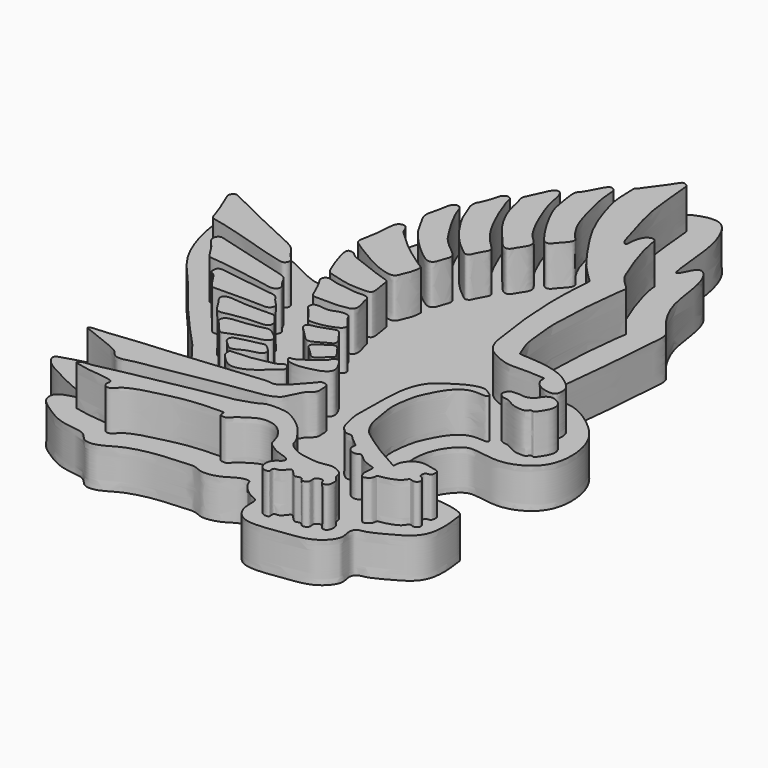
from build123d import *

# Parameters (mm, degrees)
F1_DEPTH     = 6.35
F3_DEPTH     = 6.35
F4_TEXT_SIZE = 5.2916666667
F5_DEPTH     = 3.175


# Not quite as in the source:
# - Text() gives the source's letters only with a copy of the font that has no kerning and outlines rounded to 1/6400 em; it was checked with that copy


with BuildPart() as f1:
    # F0 (on Top) → F1 (new body)
    with BuildSketch(Plane.XY):
        with BuildLine():
            add(Edge.make_bspline(
                [(-27.4553894997, -3.6191386171), (-26.8148858623, -4.1102651007), (-23.852993645, -3.5244667119), (-19.6757928123, -5.9814521208), (-16.3620676812, -9.2249197931), (-15.134802647, -13.3455814251), (-15.4166893319, -17.3130262849), (-17.4067311544, -20.0657025566), (-21.3949835552, -21.7431024541), (-25.6721295645, -20.6423826225), (-27.4943653261, -21.014570957), (-30.1702119684, -24.3150717379), (-30.2802703422, -29.5472485721), (-28.6378266919, -32.5947393842), (-24.4948659431, -36.2971740537), (-24.6097722846, -35.7640374591), (-22.7256148355, -34.3537072998), (-19.9838857156, -34.17260274), (-16.1665206622, -35.0662995786), (-16.01876004, -36.4181670777), (-15.67674916, -38.8146980995), (-15.8825278444, -43.0204957049), (-19.6794449856, -45.1478855127), (-22.3966423214, -46.5653511476), (-23.8193292554, -46.5918135896), (-24.3315319164, -47.8680905745), (-23.4823198149, -49.6082898374), (-25.9797320865, -52.64472308), (-30.6284736045, -52.9784109562), (-36.6825719823, -54.1169835226), (-38.7262257761, -50.7227346389), (-38.178485687, -48.1870624493), (-39.7768169823, -47.9738357147), (-42.0747997432, -45.9266069405), (-42.1528829746, -44.5168254865), (-44.2010819037, -44.9708731179), (-45.6685747061, -46.265967929), (-48.5542453701, -46.8428397062), (-49.8489739788, -45.940550258), (-51.6228374129, -46.0511790356), (-56.146626449, -46.3052263779), (-60.5609141609, -47.3991105071), (-62.9381972186, -49.2267616876), (-65.4295923454, -49.2927904494), (-66.3402420064, -47.2115411588), (-70.4619376248, -47.3761151768), (-73.6939821084, -45.2279395024), (-75.9213213355, -43.7444153615), (-76.1391517056, -41.6983734099), (-74.4737968942, -40.9017717278), (-72.7440822061, -40.6254899438), (-73.5010226256, -39.3395362954), (-76.0868419464, -38.415358059), (-78.7466419035, -37.0181314637), (-81.509071455, -35.6219927692), (-82.5651907032, -33.8226246448), (-80.9983905465, -33.3037701567), (-77.5024751636, -32.254660401), (-72.4511735406, -31.4168103779), (-67.3716768937, -30.6242442583), (-61.6508699498, -30.1812119822), (-61.7417475551, -29.6456508926), (-63.6792790879, -28.7025388346), (-66.8723911155, -26.0842687498), (-70.2278120042, -20.9467909755), (-73.9013952401, -17.3307431856), (-77.8419546016, -12.7167214029), (-81.8910703294, -7.3715338731), (-86.6721431792, -2.5965176686), (-88.9036740965, 4.918714181), (-88.8127902387, 8.3216580903), (-86.3142483502, 9.6224031711), (-82.2236034861, 8.0177620985), (-77.3124733662, 5.7624700254), (-72.4527478379, 3.3357110176), (-69.2384876898, 1.8166866233), (-67.2700148696, 2.21250367), (-68.0858159555, 5.2728469546), (-66.9871767241, 15.5792365266), (-62.6319303168, 26.3777930058), (-55.6842905211, 34.5100271747), (-49.290789682, 41.2499895243), (-44.4136194721, 45.7688665862), (-40.2069498195, 46.4674079992), (-38.2032900339, 44.1761388267), (-36.5613960949, 39.3943156931), (-36.303897104, 31.6116558315), (-35.3991681833, 32.1978806145), (-34.3181016042, 35.4947992226), (-31.4725448683, 32.2556409674), (-31.4109800539, 25.001298032), (-28.3660116525, 20.3349730668), (-26.8568790063, 18.7990546265), (-26.1921148547, 17.6879870326), (-26.6966478826, 14.2454097072), (-26.9886248875, 7.4933321266), (-27.9702700223, 0.0059592108), (-28.0853048722, -3.1361310215), (-27.4553894997, -3.6191386171)],
                knots=[0, 0, 0, 0, 0.0102621916, 0.0227218197, 0.0348262991, 0.0463747981, 0.057411536, 0.0674874786, 0.0790393719, 0.090657883, 0.0979966659, 0.1091456486, 0.121681532, 0.1330577825, 0.145274568, 0.1473172661, 0.1553303702, 0.165306988, 0.1759270057, 0.1817842271, 0.1905518788, 0.2017402263, 0.2132683224, 0.223194592, 0.2294367437, 0.2352939745, 0.242669919, 0.2528415109, 0.2653015886, 0.2788250284, 0.289029544, 0.2972399684, 0.3036406236, 0.3134592332, 0.3193121223, 0.3264488909, 0.3347261295, 0.344060323, 0.3508013577, 0.358032055, 0.3701207994, 0.3823246692, 0.3920357684, 0.4001190012, 0.407742519, 0.4186987314, 0.4299985352, 0.4390559444, 0.4461638099, 0.4536063147, 0.4602665683, 0.4656710985, 0.475032247, 0.485122963, 0.4951966568, 0.5021544279, 0.5082212727, 0.5190921769, 0.53186903, 0.5456635737, 0.5583206343, 0.5606866931, 0.5684030459, 0.5801350725, 0.5941202994, 0.6070219287, 0.620874169, 0.6354901951, 0.6503437704, 0.6660305311, 0.6758093578, 0.684132537, 0.695689388, 0.709120467, 0.7224849194, 0.7330496428, 0.7395731425, 0.7483200548, 0.766449771, 0.7860532177, 0.8045068132, 0.8218530155, 0.8363389009, 0.8470660296, 0.855966461, 0.8695152216, 0.8842974, 0.8878355848, 0.8969074862, 0.9060257583, 0.9216498602, 0.9348900886, 0.9428624087, 0.9487836087, 0.9588296365, 0.9738768003, 0.9899074542, 1, 1, 1, 1], degree=3))
        make_face()
    extrude(amount=-F1_DEPTH)

    # F2 (on Top) → F3 (join)
    with BuildSketch(Plane.XY):
        with BuildLine():
            add(Edge.make_bspline(
                [(-51.0431602597, -25.3127384931), (-51.2745821125, -25.3537660897), (-51.585693366, -25.239255998), (-51.5787417257, -25.7320025318), (-51.0000741928, -26.1592512167), (-50.2883419739, -26.4066127401), (-48.816850342, -26.3642354669), (-47.1832319042, -25.99359218), (-45.9112985427, -25.6087092918), (-45.0409266593, -24.8374675899), (-45.1042588573, -23.987436465), (-45.5408711668, -23.096610778), (-46.0647671328, -22.2476824891), (-46.4320555822, -21.9090460337), (-47.2162788837, -22.1575464864), (-47.2721777337, -22.7723006473), (-48.1069895995, -23.3821565507), (-49.2131278523, -24.2342290478), (-50.5653879125, -25.2280366774), (-51.0431602597, -25.3127384931)],
                knots=[0, 0, 0, 0, 0.0424248728, 0.0759988598, 0.1263997239, 0.1793440747, 0.252698589, 0.3328922948, 0.4037825364, 0.4660464316, 0.5191360524, 0.580846145, 0.6417531109, 0.6825286994, 0.7324827408, 0.7773888863, 0.8363898914, 0.9124134958, 1, 1, 1, 1], degree=3))
        make_face()
        with BuildLine():
            add(Edge.make_bspline(
                [(-50.4528097808, -22.5943885744), (-50.2009072172, -22.852652467), (-49.8842219204, -23.2714485333), (-49.3902502199, -23.4402195481), (-48.8550456144, -23.2750659834), (-48.2201713559, -22.5730329172), (-47.8716591404, -22.1185440384), (-47.41584488, -21.9220884176), (-47.1480308463, -21.436422456), (-47.8219759131, -20.5732866948), (-48.4205290406, -19.6615883887), (-48.9040339159, -19.2422247347), (-49.4735887631, -19.2412667677), (-51.0267468162, -20.4093166766), (-51.5230657887, -20.649471132), (-51.7808013374, -21.241737038), (-51.4194166847, -21.7362188103), (-50.757488413, -22.2820158521), (-50.4528097808, -22.5943885744)],
                knots=[0, 0, 0, 0, 0.0691757926, 0.118099141, 0.1706462329, 0.2412938083, 0.296871049, 0.3464913425, 0.3942791216, 0.468050598, 0.5464186234, 0.6011921627, 0.6531642032, 0.7537243571, 0.8100496669, 0.8621720635, 0.9163311974, 1, 1, 1, 1], degree=3))
        make_face()
        with BuildLine():
            add(Edge.make_bspline(
                [(-54.0498159826, -16.6909024119), (-54.4309451093, -16.7886579144), (-54.9236907464, -16.8100525559), (-55.4841457374, -17.150954382), (-55.5687185192, -17.7308079959), (-54.7835864349, -18.4822947196), (-53.6163201448, -19.6962753946), (-52.9839069298, -20.2793928352), (-52.3259906358, -20.3910920539), (-51.2503700733, -19.766276845), (-50.1447575111, -19.0834435117), (-49.5010374752, -18.9237958819), (-49.5203954014, -18.1112409278), (-50.1180495337, -17.3842322229), (-50.8593436979, -16.2880320165), (-51.2832647159, -15.8181698872), (-52.1847054864, -16.0003921099), (-53.4853314458, -16.5461182281), (-54.0498159826, -16.6909024119)],
                knots=[0, 0, 0, 0, 0.0623430111, 0.110971064, 0.1547311245, 0.2209242764, 0.306790441, 0.3657968767, 0.4145757926, 0.4865400119, 0.5618634321, 0.6100527431, 0.6615361337, 0.7258796456, 0.8007919939, 0.8486138498, 0.9076647171, 1, 1, 1, 1], degree=3))
        make_face()
        with BuildLine():
            add(Edge.make_bspline(
                [(-57.7154718339, -13.8489920646), (-57.4426548223, -14.1389097227), (-56.9641719318, -14.8565380209), (-56.286049579, -15.6886598531), (-55.9632417335, -16.0690516764), (-55.4678742171, -16.0825902786), (-53.8389666291, -16.0072877773), (-52.1807885496, -15.4218217794), (-51.3527076318, -14.9966475892), (-51.0961358405, -14.3577967622), (-51.5292296243, -13.8161515471), (-52.5457778427, -12.6549920363), (-52.7339673069, -11.9861971107), (-53.2393376369, -11.7540324128), (-54.2740386114, -11.6999497685), (-55.2828903014, -12.1988716378), (-56.294745799, -12.3544712206), (-57.359318583, -12.0967884211), (-58.1195223365, -12.2280027722), (-58.3442230508, -12.618076184), (-58.3730450927, -13.2826742755), (-57.9384009706, -13.6120893405), (-57.7154718339, -13.8489920646)],
                knots=[0, 0, 0, 0, 0.0607684619, 0.1166630656, 0.1521353154, 0.1872881217, 0.2557371584, 0.3285500365, 0.3791100111, 0.4186571539, 0.4619952422, 0.5291338699, 0.5726437839, 0.6097809741, 0.6635049593, 0.7205178734, 0.774489611, 0.8309049622, 0.8758032687, 0.9095722481, 0.950343783, 1, 1, 1, 1], degree=3))
        make_face()
        with BuildLine():
            add(Edge.make_bspline(
                [(-60.7358627021, -8.3436481655), (-60.5109025038, -8.8366568045), (-60.0222166665, -9.929884189), (-59.7570486348, -10.4844665724), (-58.9535402781, -10.6414034882), (-56.8626474343, -10.5041612494), (-55.6637065415, -10.6341358809), (-54.7588632897, -10.3865299306), (-53.9212650186, -10.3516184605), (-53.3479837532, -10.0031467426), (-53.3797547819, -8.7030940872), (-53.8434332345, -7.7117374992), (-53.8591402127, -6.9498398962), (-54.4305145001, -6.3020606164), (-56.0589847258, -6.5427869114), (-57.6440529799, -6.2479909036), (-59.3693243668, -6.0882031906), (-60.4773564804, -5.7059013677), (-61.1720251234, -5.4724937862), (-61.7435067891, -5.9118030363), (-61.8360537136, -6.5333694945), (-61.1522655527, -7.4480877708), (-60.9094500005, -7.9632251468), (-60.7358627021, -8.3436481655)],
                knots=[0, 0, 0, 0, 0.0624029211, 0.0974424366, 0.1372974836, 0.2058511483, 0.2583779573, 0.3030843904, 0.3456217278, 0.3807091631, 0.4320737739, 0.4821055108, 0.5218767272, 0.5611719847, 0.6194538937, 0.680689788, 0.7425669549, 0.793462225, 0.8318720338, 0.868564241, 0.9035233534, 0.9518476843, 1, 1, 1, 1], degree=3))
        make_face()
        with BuildLine():
            add(Edge.make_bspline(
                [(-63.1658956409, -1.7125232844), (-63.0045333751, -2.1921836237), (-62.4267597088, -3.619248892), (-62.0076478412, -4.3340511705), (-60.5316804198, -4.7342371742), (-58.3200695619, -5.3290594722), (-56.8862224099, -5.3724035497), (-55.1673104854, -5.443421827), (-54.3485208479, -5.1358791957), (-54.6817931828, -3.3548648601), (-54.864479756, -2.182940092), (-54.9692438631, -1.5676601204), (-56.3391111992, -1.2358353906), (-58.7053830333, -0.3204373165), (-60.8115823361, 0.4237868214), (-62.3934344299, 1.0489225409), (-62.8427436767, 1.7102418304), (-63.6170293643, 1.8040869196), (-63.9838731163, 1.6413681894), (-63.9428352401, 0.5020270597), (-63.3329459418, -1.0564756941), (-63.2621516745, -1.4263956598), (-63.1658956409, -1.7125232844)],
                knots=[0, 0, 0, 0, 0.0632553349, 0.1035080117, 0.1567836407, 0.2245909001, 0.2797039683, 0.3373897643, 0.3733866441, 0.4306452931, 0.480800148, 0.5119031271, 0.5615171308, 0.6339424884, 0.7023298543, 0.7588686609, 0.7974842832, 0.8347087637, 0.8591793167, 0.9047103225, 0.9622668433, 1, 1, 1, 1], degree=3))
        make_face()
        with BuildLine():
            add(Edge.make_bspline(
                [(-54.5166023076, 1.4176972909), (-54.6447443239, 1.0994388626), (-54.8698592937, 0.2716580084), (-55.5827005827, -0.2034733354), (-57.5127285564, 0.3038740625), (-59.4111238997, 1.1389104479), (-61.6868451024, 2.498020546), (-63.5273637309, 3.6024866333), (-64.2630764338, 4.1697785139), (-64.6025305916, 4.682970505), (-64.1201272309, 6.4661454363), (-63.8888361785, 8.6367543167), (-63.8404456098, 10.0627233024), (-63.6938059845, 10.9044395082), (-63.1964883809, 11.4137262798), (-62.4477548249, 11.4092981949), (-62.0200031326, 10.9287249345), (-61.788630202, 9.988860788), (-60.6421140061, 8.9994838577), (-58.2929077591, 6.7758939232), (-56.4615499088, 5.5470369783), (-54.2249516192, 3.943826605), (-53.8537274399, 3.860001145), (-54.1412079286, 2.0873732774), (-54.4060345119, 1.6923077104), (-54.5166023076, 1.4176972909)],
                knots=[0, 0, 0, 0, 0.0403213228, 0.0722907996, 0.123225953, 0.1786009007, 0.2402506999, 0.295383211, 0.3301347634, 0.3567284474, 0.406328799, 0.4634682132, 0.5080869031, 0.5417299103, 0.5717362827, 0.6021603181, 0.6307636117, 0.6660244815, 0.7118570167, 0.7785806429, 0.8384723649, 0.8982011422, 0.918092635, 0.9652086028, 1, 1, 1, 1], degree=3))
        make_face()
        with BuildLine():
            add(Edge.make_bspline(
                [(-53.1711541116, 7.1701635607), (-53.3105781169, 6.7492806406), (-53.4716730845, 5.9789526739), (-54.2863918399, 5.6005413816), (-55.4231005052, 6.2283311505), (-57.2882570655, 7.7624896831), (-59.5468859643, 10.0709520788), (-60.6654709352, 11.6820484836), (-61.7566180282, 13.7522765324), (-62.3966302917, 14.8764981582), (-62.3275485786, 15.977989267), (-61.9880298763, 16.9363475846), (-61.7731718938, 18.4349866598), (-61.569983331, 19.2516531435), (-61.0211940861, 19.7970319664), (-60.2066459209, 19.5275052108), (-59.9675942575, 18.7598000322), (-59.6092806702, 17.7060062264), (-58.3475878373, 15.2595831608), (-57.3093597118, 13.6623655769), (-56.1212070678, 11.63494563), (-54.39603909, 10.1563411757), (-53.0426019954, 9.1157164841), (-52.697914576, 8.3116263071), (-53.0320326557, 7.5901331671), (-53.1711541116, 7.1701635607)],
                knots=[0, 0, 0, 0, 0.039898997, 0.0702664358, 0.1092829888, 0.1666472165, 0.2319081805, 0.2837228223, 0.3386738763, 0.3797090762, 0.4160458165, 0.4532174902, 0.4977869395, 0.5312683359, 0.5606193333, 0.5910624073, 0.6219561444, 0.6605316435, 0.720323481, 0.7717601497, 0.8266202781, 0.882147647, 0.9288142546, 0.9601875836, 1, 1, 1, 1], degree=3))
        make_face()
        with BuildLine():
            add(Edge.make_bspline(
                [(-51.0917045176, 10.9392181039), (-50.9316985491, 11.3158911058), (-50.3528916686, 12.2805013852), (-50.1531429412, 12.6678430146), (-50.1812438653, 13.2395001883), (-50.7664969895, 13.7285995148), (-52.5108285766, 15.5683909941), (-54.0314576577, 17.9494110834), (-55.3060962907, 20.6428028672), (-56.4803985508, 23.6078114587), (-56.7334668006, 24.5797465807), (-56.7771196516, 25.1520674835), (-57.3520138011, 25.5892177215), (-58.216930852, 25.3002126115), (-58.3961059888, 24.1185147938), (-59.1377946686, 22.10096233), (-59.5553529504, 21.6305186663), (-59.5625931359, 20.534293305), (-59.0133823443, 19.5552161164), (-58.4417468898, 17.5616656282), (-56.8585294675, 15.0999632533), (-55.3395474196, 12.9655536672), (-53.569806434, 11.263160302), (-52.434838729, 10.4501372633), (-51.9004632146, 9.9596016167), (-51.2275285866, 10.4246897047), (-51.1889013683, 10.7104052049), (-51.0917045176, 10.9392181039)],
                knots=[0, 0, 0, 0, 0.0428191915, 0.0665158463, 0.0901826796, 0.1192645229, 0.1738998829, 0.2330867527, 0.2943581485, 0.3560382157, 0.3899960048, 0.4148468355, 0.4421371427, 0.4714925245, 0.5092073668, 0.5598807532, 0.5874582961, 0.6214236717, 0.6580905013, 0.7075789677, 0.7672274593, 0.8242719642, 0.8786200138, 0.9195011783, 0.9464068898, 0.9739891543, 1, 1, 1, 1], degree=3))
        make_face()
        with BuildLine():
            add(Edge.make_bspline(
                [(-47.9384362698, 15.4462410137), (-48.1485071319, 15.0888367792), (-48.439799129, 14.4005355663), (-49.5143881239, 14.4486574045), (-50.5872523186, 15.9064331362), (-52.7048998917, 18.1192732527), (-55.0535786663, 22.0368695313), (-55.5554723592, 25.3791421715), (-56.047950592, 26.3482300709), (-55.1830697963, 27.8480265522), (-54.4659959127, 29.8143455459), (-53.8584459064, 30.5158066731), (-53.1022762667, 30.581119463), (-52.5234780041, 29.3820377371), (-52.2673493499, 27.3033143389), (-51.3487014244, 24.7516881437), (-49.9692488311, 21.3690426082), (-48.4465691577, 18.9102443266), (-47.2231523777, 18.0050783015), (-47.0024361702, 17.2741434341), (-47.1933450462, 16.4949970442), (-47.708548397, 15.8373609357), (-47.9384362698, 15.4462410137)],
                knots=[0, 0, 0, 0, 0.039865054, 0.0738579514, 0.1231907968, 0.1907245817, 0.2736975541, 0.342631572, 0.3794403252, 0.4280645022, 0.4843416426, 0.5196037397, 0.5482098592, 0.589097779, 0.644576485, 0.7078489474, 0.7817048357, 0.8468647205, 0.8922445629, 0.9233351121, 0.9563742807, 1, 1, 1, 1], degree=3))
        make_face()
        with BuildLine():
            add(Edge.make_bspline(
                [(-44.8181889951, 19.6065697819), (-45.0892064683, 19.2871625125), (-45.3788242436, 18.7999570147), (-46.2986300849, 18.590227551), (-47.4578400977, 20.2381493905), (-48.8852804579, 22.3426059612), (-50.8161913432, 25.9981887098), (-51.1444078282, 27.884796994), (-51.8268805321, 31.5411972258), (-51.0618173958, 32.0335731457), (-50.0871851427, 33.9191341711), (-49.5800350058, 34.9476354883), (-49.0395552817, 35.5252647073), (-48.0908482922, 35.1087779939), (-48.1312390451, 33.8118591772), (-47.792653536, 31.1049486779), (-47.0194097064, 28.4879754833), (-46.0895843554, 24.6840873365), (-44.1677175413, 22.1645527023), (-43.6017539823, 21.6738521255), (-43.5545785906, 20.8678150492), (-44.4563897318, 20.0329678049), (-44.8181889951, 19.6065697819)],
                knots=[0, 0, 0, 0, 0.0378274782, 0.0691585245, 0.1195601458, 0.1829731268, 0.2583107602, 0.3149733325, 0.3842953787, 0.4185585686, 0.4729611357, 0.5149839133, 0.5455084659, 0.578607853, 0.6197428268, 0.6820513078, 0.7458440771, 0.8220643302, 0.8882718996, 0.9190368084, 0.9495015817, 1, 1, 1, 1], degree=3))
        make_face()
        with BuildLine():
            add(Edge.make_bspline(
                [(-52.1277524531, -27.7087949216), (-51.8088840319, -27.6149246016), (-51.286925511, -27.4192252053), (-50.9870676499, -27.0151117761), (-50.3096205755, -27.1869428315), (-49.8486741782, -28.1034559834), (-50.8239688554, -28.915458337), (-53.0422379923, -30.8232362152), (-54.5368178641, -31.505509584), (-56.3342580058, -31.7646219494), (-57.8074216971, -30.2967440914), (-58.5308978238, -29.5099387288), (-58.5333976199, -28.4641574981), (-58.0577588336, -28.5419980378), (-57.005444184, -28.4553344204), (-55.4182671766, -28.4078400516), (-53.4163705845, -28.0067200418), (-52.5125475895, -27.8220731274), (-52.1277524531, -27.7087949216)],
                knots=[0, 0, 0, 0, 0.0543149208, 0.0920882672, 0.1357996319, 0.1873570917, 0.2479667751, 0.3467624855, 0.4217089292, 0.4949345576, 0.5752045882, 0.6361262063, 0.6872002987, 0.7200634138, 0.7782354761, 0.8522042876, 0.9344553553, 1, 1, 1, 1], degree=3))
        make_face()
        with BuildLine():
            add(Edge.make_bspline(
                [(-59.1037757695, -27.8701167554), (-59.3867114578, -27.7586753043), (-59.9015092741, -27.1582175687), (-60.752400481, -26.5310875516), (-60.6486679325, -25.5186310355), (-59.7587590572, -25.3350527773), (-58.0999296109, -24.843394082), (-56.6078943641, -24.6179665266), (-56.0142146092, -24.335954542), (-54.8437192915, -25.3786490842), (-54.6154403266, -26.0301054732), (-55.0249652733, -26.7552581276), (-56.8976626709, -26.9520600961), (-58.2138886704, -27.8513727568), (-58.85678463, -27.9674005274), (-59.1037757695, -27.8701167554)],
                knots=[0, 0, 0, 0, 0.0764864722, 0.1521062383, 0.2170449898, 0.2828926781, 0.3829175026, 0.473739006, 0.5298584413, 0.6185554221, 0.6785568114, 0.7380386801, 0.8382194979, 0.9332304771, 1, 1, 1, 1], degree=3))
        make_face()
        with BuildLine():
            add(Edge.make_bspline(
                [(-64.1955733299, -23.5584191978), (-64.4168101868, -23.3225329439), (-64.8914748812, -22.8895621988), (-64.6162161632, -21.9752148969), (-63.5384869306, -21.639683951), (-62.0631338553, -21.6102629156), (-59.5317277557, -21.2198383227), (-58.2944643813, -20.805447507), (-57.5752089731, -21.2453764724), (-56.275804026, -22.2599392976), (-56.188069735, -23.0564824809), (-57.0851128872, -23.7105777497), (-58.2721813874, -23.7969972815), (-60.4757327663, -24.5644636684), (-61.9118511863, -25.1201866516), (-62.6279019718, -25.4661083664), (-63.5162139191, -24.3799194723), (-63.9494881965, -23.8207990792), (-64.1955733299, -23.5584191978)],
                knots=[0, 0, 0, 0, 0.0542836285, 0.1034632979, 0.1604990261, 0.2312516689, 0.323195176, 0.3857590257, 0.4364446556, 0.5086048249, 0.5544493793, 0.6095763308, 0.6724148373, 0.7599936256, 0.8313677159, 0.8764142381, 0.9396194912, 1, 1, 1, 1], degree=3))
        make_face()
        with BuildLine():
            add(Edge.make_bspline(
                [(-59.4865120947, -18.425444141), (-59.2638501523, -18.6830200711), (-58.8257997499, -19.0313878599), (-58.8116014315, -20.0025863892), (-59.3794496569, -20.4197684226), (-60.8016950369, -20.2884110893), (-64.4641465023, -20.7320199747), (-65.7044642864, -21.1557047885), (-66.7138447348, -21.0567343718), (-67.4807513994, -19.4746651997), (-68.309721875, -18.5362976168), (-68.4801477188, -17.8282118041), (-67.8498206622, -17.1734034611), (-65.9742048578, -17.5155911769), (-63.172923641, -17.6280361999), (-60.7868338767, -17.5369060919), (-60.143848462, -17.4995899714), (-59.7294264447, -18.1444401719), (-59.4865120947, -18.425444141)],
                knots=[0, 0, 0, 0, 0.0520802351, 0.1018697119, 0.1426877185, 0.2079163619, 0.31431348, 0.3777797851, 0.4273616376, 0.4986611868, 0.5612411578, 0.6041474294, 0.6496069169, 0.7228084543, 0.8188129076, 0.9024515806, 0.9431827625, 1, 1, 1, 1], degree=3))
        make_face()
        with BuildLine():
            add(Edge.make_bspline(
                [(-62.6528635621, -14.2897320911), (-62.3977079997, -14.6054204859), (-61.8006268013, -15.1674059642), (-61.497322134, -15.6402146615), (-61.8927338613, -16.5733610994), (-63.5119533205, -16.4274544566), (-67.6943494865, -16.4249644458), (-70.5294653786, -16.4981483154), (-70.9313768732, -16.4816516671), (-71.7635540579, -15.5852705442), (-72.849471562, -13.5195999757), (-73.7076458282, -13.524291081), (-73.6746109316, -12.3686058372), (-73.3505191838, -11.9918400504), (-72.0982646784, -12.0703922949), (-70.1896615181, -12.4356531572), (-67.546822934, -12.732640641), (-65.0660478183, -13.2275666342), (-63.838902823, -13.2188493763), (-63.1298621483, -13.555889556), (-62.8678978928, -14.0236832462), (-62.6528635621, -14.2897320911)],
                knots=[0, 0, 0, 0, 0.0509343677, 0.0839290619, 0.123384639, 0.1779115246, 0.2754749073, 0.3509697989, 0.3766312536, 0.4260584754, 0.4957413496, 0.5323748479, 0.5768002726, 0.6067240334, 0.6551090129, 0.7199823636, 0.7960430866, 0.8692766927, 0.9190421853, 0.9570746663, 1, 1, 1, 1], degree=3))
        make_face()
        with BuildLine():
            add(Edge.make_bspline(
                [(-66.8619051576, -11.7525765672), (-66.2701691893, -11.8815024837), (-65.3107184009, -12.1282045646), (-64.3701470806, -11.965649363), (-64.0147434413, -11.0028691337), (-64.8343045592, -10.3881857837), (-65.2893910164, -9.1562926335), (-66.0574748292, -8.5663895177), (-69.1944647731, -7.8308505795), (-75.1531706585, -6.1115127541), (-77.8193287156, -5.4869397053), (-78.4281626618, -5.2018445839), (-79.1176797749, -5.6199690375), (-79.1043339929, -6.7076426649), (-77.8175012481, -7.8023778893), (-76.6374502223, -9.9047340902), (-76.1984675184, -10.4337264037), (-75.0251424462, -10.4498435338), (-72.246409815, -10.8265705579), (-69.1980007336, -11.3113787566), (-67.5668439912, -11.5989863005), (-66.8619051576, -11.7525765672)],
                knots=[0, 0, 0, 0, 0.0529600871, 0.0907774368, 0.127154733, 0.1671327934, 0.2135701099, 0.2515924569, 0.3245815065, 0.4309471023, 0.497779314, 0.5285956785, 0.5617547862, 0.600551643, 0.6550121906, 0.7191381514, 0.7512139051, 0.7929947687, 0.862844648, 0.9369083105, 1, 1, 1, 1], degree=3))
        make_face()
        with BuildLine():
            add(Edge.make_bspline(
                [(-71.2615996599, -5.1090423949), (-70.4631008902, -5.3435177553), (-69.4632372964, -5.6107758644), (-68.834167347, -5.773173774), (-67.9885293739, -5.9013314837), (-67.5317600076, -4.8434733445), (-68.4765070079, -4.0590965262), (-69.6106289121, -2.375855799), (-70.3916346128, -1.617181223), (-73.5830397405, -0.2065595287), (-78.1218816729, 1.9252524168), (-81.2714985369, 3.4578896703), (-83.5852417436, 4.630767153), (-84.2986240097, 4.9463594455), (-84.9228571918, 4.2332506087), (-84.6636907092, 3.5702475801), (-84.2535929979, 2.5554044711), (-83.1602850664, 0.0962207701), (-82.6579706456, -2.0007666105), (-81.6558591101, -2.0949385291), (-79.0593230325, -2.7504954116), (-75.565828532, -3.7699971794), (-72.4777596098, -4.7519228183), (-71.2615996599, -5.1090423949)],
                knots=[0, 0, 0, 0, 0.0490835053, 0.077286376, 0.1073599005, 0.1397253549, 0.1776905971, 0.2277843546, 0.2644362885, 0.329069714, 0.4101177168, 0.4781661723, 0.5338987714, 0.5623478196, 0.592797959, 0.6208057773, 0.6576135469, 0.7172331237, 0.7670354796, 0.7987002829, 0.85530244, 0.925242974, 1, 1, 1, 1], degree=3))
        make_face()
        with BuildLine():
            add(Edge.make_bspline(
                [(-51.9071891904, -32.1571677923), (-51.07455096, -32.0522214858), (-49.8508497488, -31.8607757627), (-48.585484399, -32.2064613342), (-47.4498958079, -31.3924545937), (-46.2316340085, -30.1807015959), (-45.4019635772, -29.075201072), (-44.6526522348, -28.4572540991), (-44.5677629795, -27.9241058538), (-43.1517542975, -27.9457279179), (-43.1723363643, -29.2827721735), (-43.0335081252, -30.4800644198), (-44.0839563087, -31.0706504058), (-44.5344768344, -31.8679549033), (-45.3309004382, -33.4034773807), (-45.6251172092, -34.2340793909), (-47.1986052903, -35.1081053146), (-49.3106441982, -35.256099549), (-51.7268238139, -35.6910002962), (-54.6552759898, -36.149485254), (-58.3143567607, -36.8672059707), (-61.7635557634, -37.5272027836), (-65.547731188, -38.0024931694), (-67.3450645438, -38.6822942639), (-68.8866973751, -38.5939279409), (-69.3541255251, -37.6602100702), (-70.7371134244, -36.8279596191), (-73.2207689511, -35.9789150064), (-74.9093391231, -35.1679894333), (-75.645559461, -34.9988560819), (-76.334361308, -34.7235488724), (-75.9351130034, -34.3431051573), (-74.1704683692, -34.3320533466), (-71.2658404476, -33.9741850223), (-67.9313063596, -33.6069991004), (-64.7567043045, -33.4221697777), (-61.8352499356, -33.0811551589), (-58.192906627, -32.7946828866), (-55.4012420138, -32.5311643445), (-52.9666556066, -32.2907036825), (-51.9071891904, -32.1571677923)],
                knots=[0, 0, 0, 0, 0.0287622861, 0.0500595835, 0.0723976459, 0.0985352731, 0.1220632318, 0.1408094789, 0.1537767949, 0.1736478494, 0.1947710594, 0.2158371373, 0.2357799534, 0.2550800426, 0.2806576396, 0.2990932637, 0.3242004299, 0.3531044377, 0.3838444966, 0.4178547131, 0.4557863335, 0.4934656892, 0.5316873657, 0.5592297799, 0.5818388488, 0.6005850959, 0.6251637633, 0.6577716167, 0.6845435817, 0.7021224475, 0.7167031512, 0.7272860171, 0.7527416706, 0.787167222, 0.8235339203, 0.8584732669, 0.8924940692, 0.9297985977, 0.9634022615, 1, 1, 1, 1], degree=3))
        make_face()
        with BuildLine():
            add(Edge.make_bspline(
                [(-57.1949258447, -42.7802577615), (-58.1706471005, -42.999529365), (-60.5710759938, -43.5315633893), (-62.9924696457, -44.5929069533), (-63.5162225887, -45.5869158783), (-64.5376439163, -45.8239589889), (-65.0969237621, -44.9727031982), (-64.6993878533, -44.1858354732), (-65.6605164974, -43.7874803259), (-67.4807971236, -43.5437612611), (-68.8502416915, -43.4996280525), (-70.7364737347, -43.0306539215), (-71.5813313627, -42.9428717034), (-71.0912718939, -42.2270145464), (-69.7035858699, -42.3030269242), (-66.8272844875, -41.5432601258), (-62.7843087235, -40.777520996), (-59.478087155, -40.1876496599), (-57.7102801843, -39.7542481777), (-53.8255911736, -38.9979511891), (-50.2211556603, -38.5203204195), (-48.3332755057, -37.9057410983), (-46.6256798803, -37.287428357), (-46.025623031, -36.7214053137), (-42.8953288623, -36.7521334164), (-41.5797634226, -37.3900552453), (-39.3953484926, -38.8468471896), (-37.9977052019, -40.6391034953), (-36.940044694, -42.1669341398), (-36.7699882452, -43.1305197641), (-36.1051134427, -43.8204415866), (-34.4553314026, -44.7319252863), (-33.1255561435, -44.867220155), (-31.5753462115, -45.1701386188), (-30.082786851, -44.9787946146), (-28.8963249158, -44.680189287), (-27.0165497879, -45.6863319545), (-27.2048031787, -46.621206143), (-26.6760591905, -47.1376853401), (-26.2413706244, -47.6436076652), (-26.2658936001, -48.7120206333), (-26.6857534859, -49.2902562708), (-27.5147939317, -49.162854106), (-27.5733542058, -48.414667587), (-28.1731194572, -48.350638569), (-28.976302893, -48.7464426891), (-28.7617595869, -49.4769467611), (-28.8396192822, -50.0034587273), (-29.8000321327, -50.3585366512), (-30.0116592842, -49.5995433477), (-30.6479008155, -49.6979391367), (-31.274889969, -49.9465623803), (-32.0132335187, -48.9389318405), (-32.6136925156, -48.4864167719), (-32.9410498055, -49.0501189193), (-33.428735821, -49.5949129844), (-33.8077290884, -49.7907480772), (-34.4598122968, -49.7258154922), (-34.5091286663, -50.33594787), (-34.3383288856, -50.8479214072), (-35.3902809782, -50.9278021838), (-36.0244854678, -50.1219927347), (-36.1988899244, -49.4341091829), (-36.0551749482, -48.4614763278), (-35.354972636, -47.8401094371), (-34.8595230338, -47.5947419356), (-34.5911212237, -46.8661691805), (-35.5908164421, -46.3976604748), (-36.7961398937, -46.1429724113), (-38.1065140173, -45.3434451971), (-39.001906767, -44.7455578311), (-39.1819075428, -43.2676039458), (-40.1309568373, -41.7174964399), (-41.4205694357, -40.6050748948), (-42.8307466311, -40.2347408849), (-44.2947314765, -40.3401171991), (-45.7394724801, -41.2631017576), (-47.0638472301, -42.1559606543), (-47.4429638572, -42.9123664834), (-48.1676869711, -42.8352436833), (-48.6677032336, -42.837977966), (-48.6563176361, -42.1489076282), (-48.7001749884, -41.8768262374), (-49.3372077722, -41.894639309), (-52.2401627341, -41.8929415625), (-55.2055216047, -42.328019157), (-56.4519703779, -42.6132950808), (-57.1949258447, -42.7802577615)],
                knots=[0, 0, 0, 0, 0.0202665824, 0.0376091016, 0.0485277873, 0.0584165759, 0.0682492227, 0.0771801548, 0.0868868262, 0.1016092147, 0.1147704607, 0.1299958151, 0.1382601255, 0.1459997507, 0.1582386005, 0.1768959026, 0.1993484437, 0.2188295302, 0.233375933, 0.2547960284, 0.2756313437, 0.2910190526, 0.3049408446, 0.3147687719, 0.3331311595, 0.346786065, 0.3638673481, 0.3805404118, 0.3950396477, 0.405280274, 0.4155706797, 0.4302125788, 0.4428809361, 0.456348821, 0.4694314343, 0.4815167203, 0.4962038559, 0.5057660553, 0.5145577298, 0.5233162401, 0.5341540869, 0.5427548482, 0.5514389702, 0.559824517, 0.5674372068, 0.5768898076, 0.5855944088, 0.5931784654, 0.6026941655, 0.6108810793, 0.6187892427, 0.627061449, 0.6388096667, 0.6472058373, 0.6549704834, 0.664306228, 0.6713779701, 0.6792311443, 0.6868701383, 0.693754476, 0.7032991915, 0.7139697239, 0.7230384489, 0.7334541272, 0.7436771734, 0.7517265916, 0.7598606894, 0.7701879091, 0.7825714762, 0.7958824119, 0.8066862725, 0.819380571, 0.8339791494, 0.8479433012, 0.8607364125, 0.8735346767, 0.8877676901, 0.9014208418, 0.910681824, 0.91939864, 0.926280249, 0.9345949135, 0.9396708238, 0.9471022735, 0.9655713817, 0.9845681662, 1, 1, 1, 1], degree=3))
        make_face()
        with BuildLine():
            add(Edge.make_bspline(
                [(-23.1154561043, -11.1026372761), (-22.9770757948, -11.3121825974), (-22.5726937171, -11.8684888596), (-21.3042722712, -12.4425378181), (-19.8685711977, -12.5053355588), (-19.4171848607, -11.9989122903), (-19.3712848192, -10.407695408), (-20.362394649, -9.3356203769), (-22.064522429, -8.0476817209), (-24.380100568, -7.202361826), (-26.7951465635, -6.8450338589), (-28.7737953004, -6.7233434052), (-29.8872020253, -6.6918173603), (-29.9459395668, -6.2520746693), (-31.1118134258, -3.9010909546), (-31.1806919327, -0.7819432959), (-31.6195412002, 1.694741284), (-31.3690159393, 5.3095411789), (-31.2834787339, 8.4853196531), (-30.8061526629, 12.3501294762), (-30.6059808649, 14.5364012275), (-30.3799279757, 15.2047669301), (-30.7401171945, 15.625636788), (-32.4637439318, 17.1237441172), (-33.2371133551, 18.9474526736), (-34.5446210925, 22.3717685395), (-35.306479304, 25.0766300566), (-35.6908777111, 26.7567941217), (-35.6345738284, 27.6323692902), (-36.4026081774, 28.0146554824), (-37.2491596113, 27.5474616067), (-37.6572128071, 26.7369011457), (-37.9224098542, 25.5140223988), (-37.8299551298, 24.8654665434), (-38.0117774429, 24.4715263101), (-38.6317699937, 24.9212663897), (-39.1194484401, 26.6713301669), (-40.0823718988, 29.855498157), (-41.0700098003, 33.4493860117), (-41.373625032, 36.8888799424), (-41.6133917297, 38.707417032), (-41.8019456952, 41.215258448), (-41.8672058106, 41.6039883771), (-42.6200852991, 42.0710233984), (-43.0744659572, 41.7464175278), (-43.8457791333, 40.3291987467), (-45.2116657854, 38.6688084629), (-46.2488611652, 37.0527076788), (-46.5816327486, 36.972250681), (-46.5182940618, 35.8909787586), (-46.4822963171, 34.3169509169), (-46.2842950993, 32.3744797415), (-45.8051817593, 30.7619604794), (-44.9418459805, 28.0104379563), (-43.5672748446, 24.7233294117), (-41.3560816, 21.3625438439), (-38.6948953242, 17.4259384745), (-36.9027308765, 15.6071944651), (-35.4277149455, 14.125948391), (-35.2285976907, 14.0245541701), (-35.3933311222, 12.7465850401), (-35.5219740372, 9.6488202802), (-35.5936194134, 6.8401052936), (-35.3302036895, 2.4430039597), (-35.1980722843, 0.7849579655), (-34.3885577394, -4.5527234689), (-34.3114764649, -5.8370889066), (-33.5932616956, -7.5302543913), (-32.4008310294, -8.6012311839), (-30.5749518802, -9.400555829), (-29.0920197536, -9.8295388458), (-27.5565036723, -9.7449656438), (-25.4849072311, -9.7521797229), (-23.6375538477, -9.8666015345), (-23.2890452545, -9.8778395941), (-23.4038902784, -10.6328529585), (-23.2272665859, -10.9333258807), (-23.1154561043, -11.1026372761)],
                knots=[0, 0, 0, 0, 0.0095863353, 0.0218001504, 0.0336521272, 0.0413311612, 0.0535664799, 0.0657766935, 0.0806132243, 0.0967185203, 0.1128367704, 0.1275542805, 0.1373764309, 0.1431327291, 0.1592210357, 0.1776381964, 0.1939230474, 0.2130920835, 0.2317394513, 0.2521316505, 0.2671479284, 0.2748541972, 0.281840225, 0.2968701634, 0.311710815, 0.3312522832, 0.3487791739, 0.3619945713, 0.3709348257, 0.3793253662, 0.388835163, 0.398638082, 0.4100730793, 0.4184078883, 0.4238041708, 0.4311775633, 0.4447848468, 0.4636403636, 0.4838118965, 0.5024775425, 0.5170619856, 0.5327574126, 0.5391611571, 0.547955982, 0.5548070296, 0.5674767575, 0.5833767549, 0.5970309402, 0.6020432352, 0.6118278844, 0.6251566221, 0.6393142026, 0.6525645323, 0.6697622793, 0.6890988649, 0.7099280341, 0.7320997503, 0.7492099518, 0.7631477115, 0.7671980942, 0.7778204988, 0.7959637423, 0.8139671788, 0.8347311796, 0.8491990565, 0.8724180491, 0.884663929, 0.897829433, 0.9108385459, 0.925205798, 0.9378334037, 0.9503184292, 0.9655839289, 0.9793136024, 0.9841034158, 0.9922542971, 1, 1, 1, 1], degree=3))
        make_face()
        with BuildLine():
            add(Edge.make_bspline(
                [(-23.1888126582, -15.1789393276), (-22.9022265225, -15.1917256604), (-22.0316280162, -15.4107151721), (-20.7754970914, -14.7890400413), (-20.4306595113, -13.7881432771), (-19.410407196, -13.1613451809), (-18.370994566, -13.6130594913), (-17.6945894369, -14.1113569836), (-17.3371837763, -15.1223363079), (-17.6414706987, -16.2478581604), (-18.6269324178, -17.6399677512), (-18.8184143018, -17.7708874574), (-19.405221843, -17.5067418895), (-19.6074623824, -18.2434328068), (-20.6187283115, -18.2123125381), (-21.7813132306, -18.1530983722), (-23.4203517308, -17.0228773584), (-24.0186374044, -17.2223883554), (-25.0933453728, -16.5674161071), (-24.8704614976, -15.7542693851), (-24.4507445794, -15.1503666337), (-23.6677640056, -15.2421692301), (-23.3804563634, -15.1703889482), (-23.1888126582, -15.1789393276)],
                knots=[0, 0, 0, 0, 0.0534760381, 0.1108477761, 0.1617721219, 0.2132985621, 0.2648864171, 0.3107741088, 0.359992256, 0.4160461755, 0.4804264172, 0.5028706739, 0.5376676871, 0.5752100168, 0.6221541454, 0.6787562031, 0.7472028616, 0.786583131, 0.8379285201, 0.8808940569, 0.922156006, 0.9642399097, 1, 1, 1, 1], degree=3))
        make_face()
        with BuildLine():
            add(Edge.make_bspline(
                [(-29.8309884965, -18.9367402345), (-29.4434195627, -18.6206952353), (-28.5579500389, -18.0603109268), (-26.6322336839, -18.1278035603), (-25.9678639002, -18.2262243304), (-25.5493449418, -17.7139163434), (-26.7128649984, -17.0885698001), (-27.3866033434, -16.5054108465), (-29.5207213069, -17.0504405625), (-31.3439361626, -18.1523699715), (-33.8637552991, -19.7340479002), (-35.0110899096, -22.4735816721), (-35.4134267407, -25.2968384532), (-35.4254357417, -31.3874640579), (-35.4681832607, -32.5196424988), (-34.8263953408, -35.5712050772), (-34.1417133277, -36.1511627313), (-33.3872352507, -36.91224708), (-32.4208561154, -36.6499126892), (-32.04357307, -37.369029653), (-30.4004253551, -38.5178485806), (-30.4134639677, -38.7446527822), (-30.5753724793, -39.3508217245), (-30.0034250198, -40.2704175741), (-28.8839829053, -40.4676663933), (-28.40421647, -39.9726524225), (-27.8334633651, -40.4076597306), (-26.9855093309, -41.3079332589), (-25.2401908495, -41.8562426585), (-24.7941707059, -41.948149973), (-24.9436935294, -43.1409235925), (-25.0255810417, -43.7921378546), (-24.536880583, -44.9088846136), (-23.7610213302, -44.5403413285), (-23.2301453534, -44.1351623274), (-23.2570085378, -43.3773241789), (-23.0555711299, -43.3177198308), (-22.1117617909, -43.2083362687), (-20.0587859763, -42.5545677331), (-19.681697712, -41.6510880185), (-19.2888980699, -41.4274409696), (-18.7865002428, -41.7959041231), (-18.1152797745, -41.482515246), (-17.9825666232, -40.814148704), (-18.5868973547, -40.1505333781), (-19.0613037447, -40.0654379915), (-19.1048071489, -39.1140451217), (-18.4977110756, -39.0141356866), (-18.0141616558, -38.9255243058), (-17.9759511017, -38.091469762), (-18.0613083374, -37.6253278875), (-19.6150840116, -37.3144632134), (-21.183951487, -36.9740943183), (-22.4518026219, -37.7252618616), (-23.3284849572, -38.8850557859), (-23.1982663735, -40.0242518557), (-23.6688891673, -39.7736620893), (-24.3157861148, -39.4574769332), (-27.2939721202, -37.6808774746), (-26.9507509483, -37.9479338131), (-30.6620792509, -35.4916813009), (-31.6198702891, -34.556915984), (-32.6678213458, -32.5977522061), (-33.0127209243, -30.2884083209), (-33.4960794914, -27.7927333208), (-33.0714978988, -25.1161505046), (-32.7760251187, -23.6515753612), (-32.0042199138, -21.9480692546), (-31.0073193948, -20.0687366728), (-30.2268334562, -19.2595339597), (-29.8309884965, -18.9367402345)],
                knots=[0, 0, 0, 0, 0.016862829, 0.0355250256, 0.0463858192, 0.0547540813, 0.0690569124, 0.0820143665, 0.1010887497, 0.1215646272, 0.1446583129, 0.1671561275, 0.191275195, 0.2240962136, 0.2402384982, 0.263225436, 0.2764076106, 0.2897164765, 0.3018902247, 0.314033896, 0.3328962294, 0.3387183516, 0.3488044614, 0.3625059585, 0.3762794855, 0.3863707016, 0.3965199156, 0.4121931976, 0.4304221339, 0.4384167264, 0.452269881, 0.4643216095, 0.4776679619, 0.4887875337, 0.5000109927, 0.5109591063, 0.5160435255, 0.5290761808, 0.5491260271, 0.5619956469, 0.5699791821, 0.5800058181, 0.5908031205, 0.6012235635, 0.6135497617, 0.6225272292, 0.6341152402, 0.6439561843, 0.6528144596, 0.6644789469, 0.6730689362, 0.6894630521, 0.7069460324, 0.7228746982, 0.7394172183, 0.7519925841, 0.7588953431, 0.7726879967, 0.7965555844, 0.7985242666, 0.8252106856, 0.8436290516, 0.8628036151, 0.883721169, 0.9056368761, 0.9277856896, 0.9443947317, 0.9628349878, 0.9827770874, 1, 1, 1, 1], degree=3))
        make_face()
    extrude(amount=F3_DEPTH)

    # F4 (on face) → F5 (cut)
    with BuildSketch(Plane(origin=(0, 0, -6.35), x_dir=(1, 0, 0), z_dir=(0, 0, -1))):
        with Locations(Location((-69.5724026214, 14.950160879), (0, 0, -130))):
            Text('R. Frisell', F4_TEXT_SIZE, font='Open Sans', font_style=FontStyle.BOLD, text_align=(TextAlign.LEFT, TextAlign.BOTTOM))
    extrude(amount=-F5_DEPTH, mode=Mode.SUBTRACT)


solid = f1.part
